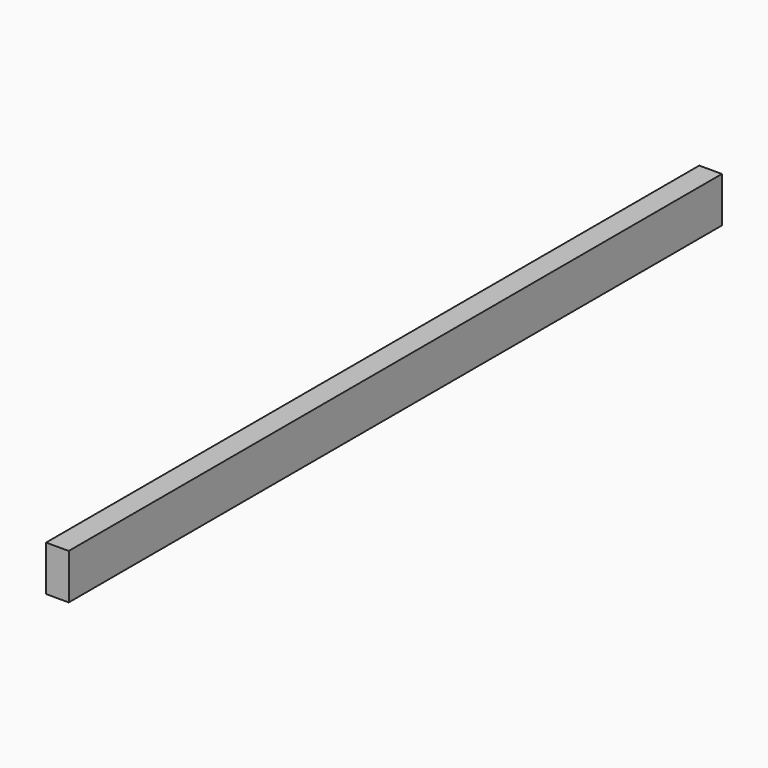
from build123d import *

# Parameters (mm, degrees)
F1_W     = 19.05
F1_H     = 38.1
F2_DEPTH = 685.8


# Not quite as in the source:
# - a variable given as a bare number and used for a length is read in inches; the dataset says mm whatever the document's units were


with BuildPart() as f2:
    # F1 (on Front) → F2 (new body)
    with BuildSketch(Plane.XZ):
        with Locations((9.525, 19.05)):
            Rectangle(F1_W, F1_H)
    extrude(amount=F2_DEPTH)


solid = f2.part
